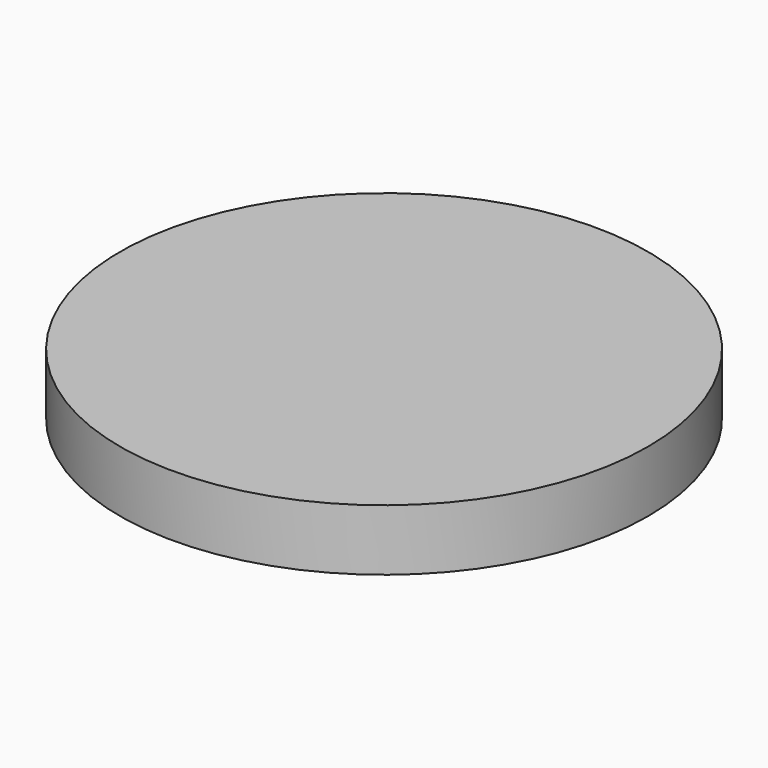
from build123d import *

# Parameters (mm, degrees)
F4_R          = 75
F5_DEPTH      = 2
F6_R          = 75
F6_R_2        = 73
F6_R_3        = 4
F7_DEPTH      = 14
F9_DEPTH      = 14
F11_DEPTH     = 14
F12_R         = 1
F13_R         = 0.5
F15_R         = 77.6
F16_DEPTH     = 2
F17_R         = 77.6
F17_R_2       = 75.6
F18_DEPTH     = 16
F20_TEXT_SIZE = 6.4814814815
F21_DEPTH     = 0.5714285714


# Not quite as in the source:
# - Text() gives the source's letters only with a copy of the font that has no kerning and outlines rounded to 1/6400 em; it was checked with that copy


with BuildPart() as f5:
    # F4 (on Top) → F5 (new body)
    with BuildSketch(Plane.XY):
        Circle(F4_R)
    extrude(amount=F5_DEPTH)

    # F6 (on face) → F7 (join)
    with BuildSketch(Plane.XY.offset(2)):
        Circle(F6_R)
        Circle(F6_R_2, mode=Mode.SUBTRACT)
        with BuildLine():
            ThreePointArc((0, 25), (-12.1833533605, 21.8303893894), (-21.2773878342, 13.1252720715))
            ThreePointArc((-21.2773878342, 13.1252720715), (-14.670401224, 8.2416315348), (-7, 5.2976271151))
            Line((-7, 5.2976271151), (-7, -13.2976271151))
            ThreePointArc((-7, -13.2976271151), (-15.9759399375, -16.9999942672), (-23.3345237792, -23.3345237792))
            ThreePointArc((-23.3345237792, -23.3345237792), (-27.5289130679, -18.1977730862), (-30.6115511413, -12.326107931))
            Line((-30.6115511413, -12.326107931), (-16.1539272827, -9.1287279932))
            Line((-16.1539272827, -9.1287279932), (-15, 0))
            Line((-15, 0), (-44.9854118741, -1.1457392878))
            ThreePointArc((-44.9854118741, -1.1457392878), (-39.1830812147, -22.1288532582), (-24.2098176006, -37.9326341261))
            Line((-24.2098176006, -37.9326341261), (-33.2161737904, -53.5321006381))
            ThreePointArc((-33.2161737904, -53.5321006381), (0, 63), (33.2161737904, -53.5321006381))
            Line((33.2161737904, -53.5321006381), (29.2138629749, -46.5998949579))
            ThreePointArc((29.2138629749, -46.5998949579), (5.0413462419, 54.7684656355), (-37.2297786461, -40.4838681695))
            Line((-37.2297786461, -40.4838681695), (-36.2297786461, -38.7518173619))
            ThreePointArc((-36.2297786461, -38.7518173619), (6.0392613317, 52.7050996789), (26.5249892064, -45.9426289757))
            Line((26.5249892064, -45.9426289757), (32.5, -56.291651246))
            ThreePointArc((32.5, -56.291651246), (36.9404281222, -53.4827520809), (41.1394772886, -50.3243818484))
            ThreePointArc((41.1394772886, -50.3243818484), (-5.24997314, 64.7876360275), (-32.5, -56.291651246))
            Line((-32.5, -56.291651246), (-21.5, -37.2390923627))
            ThreePointArc((-21.5, -37.2390923627), (-36.4480947036, -22.8152666536), (-42.8904719342, -3.0671513264))
            Line((-42.8904719342, -3.0671513264), (-17.2799239096, -2.0885751049))
            Line((-17.2799239096, -2.0885751049), (-17.9614515484, -7.4801457245))
            Line((-17.9614515484, -7.4801457245), (-33.2706082951, -10.8658466616))
            ThreePointArc((-33.2706082951, -10.8658466616), (-25.2618760789, -24.224731515), (-12.2502696285, -32.7861387484))
            Line((-12.2502696285, -32.7861387484), (-12.2502696285, -41.2180894029))
            Line((-12.2502696285, -41.2180894029), (-23.4528274088, -60.6214886532))
            Line((-23.4528274088, -60.6214886532), (-21.5766696606, -61.3143321448))
            Line((-21.5766696606, -61.3143321448), (-10.2502696285, -41.7604115466))
            Line((-10.2502696285, -41.7604115466), (-10.2502696285, -31.3676899459))
            ThreePointArc((-10.2502696285, -31.3676899459), (-16.4059499296, -28.6329322094), (-21.878104727, -24.7052329184))
            ThreePointArc((-21.878104727, -24.7052329184), (0, -14.4807088269), (21.878104727, -24.7052329184))
            ThreePointArc((21.878104727, -24.7052329184), (11.2299513945, -31.0304397596), (-1, -32.9848450049))
            Line((-1, -32.9848450049), (-1, -42.9883705204))
            Line((-1, -42.9883705204), (-11.5766696606, -63.9607748512))
            ThreePointArc((-11.5766696606, -63.9607748512), (0, -65), (11.5766696606, -63.9607748512))
            Line((11.5766696606, -63.9607748512), (1, -42.9883705204))
            Line((1, -42.9883705204), (1, -34.9857113691))
            ThreePointArc((1, -34.9857113691), (24.0039150578, -25.4717895307), (34.8648899176, -3.0723689616))
            Line((34.8648899176, -3.0723689616), (15, 0))
            Line((15, 0), (15, -9.2013707102))
            Line((15, -9.2013707102), (21.8124581524, -12.3780721176))
            Line((21.8124581524, -12.3780721176), (22.6576946759, -10.5654565435))
            Line((22.6576946759, -10.5654565435), (17, -7.9272301886))
            Line((17, -7.9272301886), (17, -2.3331059175))
            Line((17, -2.3331059175), (32.6557043977, -4.7544684553))
            ThreePointArc((32.6557043977, -4.7544684553), (29.496288356, -14.797600252), (23.3345237792, -23.3345237792))
            ThreePointArc((23.3345237792, -23.3345237792), (15.9759399375, -16.9999942672), (7, -13.2976271151))
            Line((7, -13.2976271151), (7, 5.2976271151))
            ThreePointArc((7, 5.2976271151), (18.2129872681, 10.5149423165), (26.4345544122, 19.7538435001))
            ThreePointArc((26.4345544122, 19.7538435001), (25.7751387842, 20.6068488773), (25.0882096241, 21.4378575855))
            ThreePointArc((25.0882096241, 21.4378575855), (16.7032782177, 11.8839781581), (5, 6.9224294318))
            Line((5, 6.9224294318), (5, -12.896329875))
            ThreePointArc((5, -12.896329875), (0, -12.4839230078), (-5, -12.896329875))
            Line((-5, -12.896329875), (-5, 6.9224294318))
            ThreePointArc((-5, 6.9224294318), (-12.2733040938, 9.2567295078), (-18.6661185979, 13.4378575855))
            ThreePointArc((-18.6661185979, 13.4378575855), (-12.615863454, 19.2312243321), (-4.8921894899, 22.4736842105))
            ThreePointArc((-4.8921894899, 22.4736842105), (2.7529888064, 13.6688601002), (0, 25))
        make_face()
        with BuildLine():
            ThreePointArc((7.8690650381, -62.5066221726), (-0.3472882895, -62.9990427772), (-8.5577133963, -62.4160679747))
            Line((-8.5577133963, -62.4160679747), (0, -45.4470379064))
            Line((0, -45.4470379064), (7.8690650381, -62.5066221726))
        make_face(mode=Mode.SUBTRACT)
        with Locations((0, 19)):
            Circle(F6_R_3, mode=Mode.SUBTRACT)
        with BuildLine():
            ThreePointArc((-31.7735687329, 8.9129304933), (-7.098729201, 32.2274424013), (25.0882096241, 21.4378575855))
            ThreePointArc((25.0882096241, 21.4378575855), (25.7751387842, 20.6068488773), (26.4345544122, 19.7538435001))
            ThreePointArc((26.4345544122, 19.7538435001), (29.6276296639, 14.5328441984), (31.8017058984, 8.8120089624))
            Line((31.8017058984, 8.8120089624), (33.8051079409, 9.0672309503))
            ThreePointArc((33.8051079409, 9.0672309503), (0.9592424635, 34.9868525863), (-33.2575000391, 10.905901666))
            Line((-33.2575000391, 10.905901666), (-41.6043850931, 10.8662385867))
            ThreePointArc((-41.6043850931, 10.8662385867), (30.6177255227, 30.1919672068), (10.2826166709, -41.7524585432))
            Line((10.2826166709, -41.7524585432), (21.5766696606, -61.3143321448))
            Line((21.5766696606, -61.3143321448), (23.4528274088, -60.6214886532))
            Line((23.4528274088, -60.6214886532), (13.2771569306, -42.9967103839))
            ThreePointArc((13.2771569306, -42.9967103839), (30.1654749403, 33.3922763768), (-44.1203135442, 8.8542607122))
            Line((-44.1203135442, 8.8542607122), (-31.7735687329, 8.9129304933))
        make_face()
    extrude(amount=F7_DEPTH)

    # F8 (on face) → F9 (cut, through all)
    with BuildSketch(Plane.XY.offset(16)):
        with BuildLine():
            Line((42.9913939556, -0.8602591182), (44.9909936745, -0.9002711702))
            ThreePointArc((44.9909936745, -0.9002711702), (44.6708560132, 5.4327362393), (43.4637102097, 11.6578683647))
            Line((43.4637102097, 11.6578683647), (41.5319897559, 11.1397408818))
            ThreePointArc((41.5319897559, 11.1397408818), (42.6854846349, 5.1912812953), (42.9913939556, -0.8602591182))
        make_face()
        with BuildLine():
            ThreePointArc((47.7867917709, -23.0374204684), (45.4027743681, -27.43880991), (42.6145352063, -31.595911108))
            Line((42.6145352063, -31.595911108), (44.1809687105, -32.7573198508))
            ThreePointArc((44.1809687105, -32.7573198508), (47.0716985182, -28.4474111056), (49.5433481038, -23.8842345213))
            Line((49.5433481038, -23.8842345213), (47.7867917709, -23.0374204684))
        make_face()
        with BuildLine():
            Line((-13.5789473684, 40.7996591697), (-17.3684210526, 52.1856105659))
            ThreePointArc((-17.3684210526, 52.1856105659), (-22.0283389578, 50.3959550238), (-26.5068037779, 48.1911750581))
            Line((-26.5068037779, 48.1911750581), (-22.6356800758, 36.5598958902))
            ThreePointArc((-22.6356800758, 36.5598958902), (-18.2309821019, 38.9439506419), (-13.5789473684, 40.7996591697))
        make_face()
    extrude(amount=-F9_DEPTH, mode=Mode.SUBTRACT)

    # F10 (on face) → F11 (join, through all)
    with BuildSketch(Plane.XY.offset(16)):
        with BuildLine():
            Line((-23.2840016559, 38.5078598067), (-25.880325819, 46.308843055))
            ThreePointArc((-25.880325819, 46.308843055), (-26.7676062562, 45.8016971837), (-27.6449525052, 45.2775530542))
            Line((-27.6449525052, 45.2775530542), (-25.0234436687, 37.4008992801))
            ThreePointArc((-25.0234436687, 37.4008992801), (-24.1600633039, 37.9643430228), (-23.2840016559, 38.5078598067))
        make_face()
        with BuildLine():
            Line((-9.1369131453, 33.7863407041), (-11.6665929676, 41.3870826289))
            ThreePointArc((-11.6665929676, 41.3870826289), (-12.6261868074, 41.1044937532), (-13.5789473684, 40.7996591697))
            Line((-13.5789473684, 40.7996591697), (-11.0526315789, 33.2090249056))
            ThreePointArc((-11.0526315789, 33.2090249056), (-10.0988985749, 33.5113748983), (-9.1369131453, 33.7863407041))
        make_face()
        with BuildLine():
            ThreePointArc((18.6383737373, 49.6680101677), (17.6986450604, 50.0105806067), (16.7526247619, 50.3353729814))
            Line((16.7526247619, 50.3353729814), (14.2105263158, 42.6973177358))
            ThreePointArc((14.2105263158, 42.6973177358), (15.1560791403, 42.3709011598), (16.0941428563, 42.0235477527))
            Line((16.0941428563, 42.0235477527), (18.6383737373, 49.6680101677))
        make_face()
    extrude(amount=-F11_DEPTH)

    # F12
    f12_edges = [f5.edges().sort_by_distance(p)[0] for p in [
        (-5, 6.922429, 9),
        (5, 6.922429, 9),
    ]]
    fillet(f12_edges, radius=F12_R)

    # F13
    f13_edges = [f5.edges().sort_by_distance(p)[0] for p in [
        (-15, 0, 9),
        (15, 0, 9),
        (-11.57667, -63.960775, 9),
        (11.57667, -63.960775, 9),
        (-21.5, -37.239092, 9),
    ]]
    fillet(f13_edges, radius=F13_R)

    # F20 (on 3pt) → F21 (cut)
    with BuildSketch(Plane(origin=(-0.3443241791, -62.4613450737, 0), x_dir=(-0.999984806, 0.0055125125, 0), z_dir=(0.0055125125, 0.999984806, 0))):
        with Locations((-5.5502748843, 6.6666666667)):
            Text('3E8', F20_TEXT_SIZE, font='Open Sans', text_align=(TextAlign.LEFT, TextAlign.BOTTOM))
    extrude(amount=-F21_DEPTH, mode=Mode.SUBTRACT)


with BuildPart() as f16:
    # F15 (on offset) → F16 (new body)
    with BuildSketch(Plane.XY.offset(16.6)):
        Circle(F15_R)
    extrude(amount=F16_DEPTH)

    # F17 (on face) → F18 (join)
    with BuildSketch(Plane(origin=(0, 0, 16.6), x_dir=(1, 0, 0), z_dir=(0, 0, -1))):
        Circle(F17_R)
        Circle(F17_R_2, mode=Mode.SUBTRACT)
    extrude(amount=F18_DEPTH)


solid = Compound([f5.part, f16.part])
